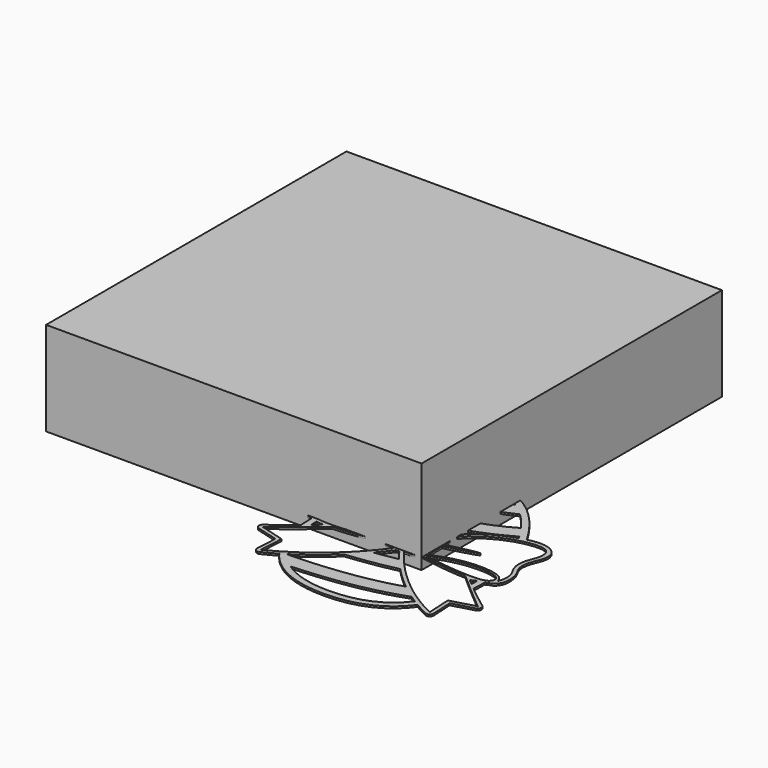
from build123d import *

# Parameters (mm, degrees)
F0_W     = 100
F0_H     = 100
F1_DEPTH = 25
F3_DEPTH = 5
F4_SCALE = 0.1


with BuildPart() as f1:
    # F0 (on Top) → F1 (new body)
    with BuildSketch(Plane.XY):
        with Locations((-50, 50)):
            Rectangle(F0_W, F0_H)
    extrude(amount=F1_DEPTH)


with BuildPart() as f3:
    # F2 (on face) → F3 (new body)
    with BuildSketch(Plane.XY.offset(25)):
        Polygon((237.0909, -93.2355584012), (234.964781, -91.1346954012), (230.904136, -88.1422674012), (225.837062, -84.3918364012), (219.722472, -79.8171774012), (212.519281, -74.3520704012), (204.186402, -67.9302914012), (194.68275, -60.4856174012), (183.967238, -51.9518264012), (171.998781, -42.2626954012), (172.36901, -37.8418454012), (172.685672, -33.4080234012), (172.949107, -28.9619434012), (173.159656, -24.5043204012), (173.317658, -20.0358694012), (173.423453, -15.5573044012), (173.477381, -11.0693414012), (173.479781, -6.5726954012), (174.402898, -6.2096524012), (175.317906, -5.8351014012), (176.224289, -5.4476604012), (177.121531, -5.0459454012), (178.009117, -4.6285744012), (178.886531, -4.1941644012), (179.753258, -3.7413324012), (180.608781, -3.2686954012), (182.202781, -2.6213224012), (184.271343, -2.0135234012), (186.723437, -1.2204044012), (189.468031, -0.0170704012), (192.414094, 1.8213725988), (195.470593, 4.5198205988), (198.5465, 8.3031655988), (201.550781, 13.3963045988), (202.989537, 16.5327435988), (204.06814, 19.5250075988), (204.83847, 22.4765135988), (205.352406, 25.4906795988), (205.661826, 28.6709235988), (205.818609, 32.1206635988), (205.874635, 35.9433185988), (205.881781, 40.2423045988), (204.442482, 53.2482925988), (201.031328, 63.6247105988), (196.627056, 72.4642385988), (192.208406, 80.8595545988), (188.754115, 89.9033395988), (187.242922, 100.6882735988), (188.653564, 114.3070345988), (193.964781, 131.8523045988), (196.39601, 137.7646815988), (199.286672, 144.9972575988), (201.940732, 153.1809505988), (203.662156, 161.9466795988), (203.754908, 170.9253615988), (201.522953, 179.7479135988), (196.270256, 188.0452555988), (187.300781, 195.4483045988), (180.359689, 198.9783925988), (172.853109, 201.4293825988), (164.869459, 202.8953655988), (156.497156, 203.4704295988), (147.824619, 203.2486655988), (138.940265, 202.3241635988), (129.932513, 200.7910135988), (120.889781, 198.7433045988), (117.827379, 204.0665255988), (114.587812, 209.4891325988), (111.207293, 214.9619195988), (107.722031, 220.4356795988), (104.168238, 225.8612045988), (100.582125, 231.1892885988), (96.999902, 236.3707245988), (93.457781, 241.3563045988), (88.759427, 247.7524355988), (84.021078, 253.9551015988), (79.243424, 259.9650875988), (74.427156, 265.7831795988), (69.572967, 271.4101615988), (64.681547, 276.8468205988), (59.753588, 282.0939395988), (54.789781, 287.1523045988), (50.867982, 290.9924065988), (46.925078, 294.7163045988), (42.961056, 298.3226405988), (38.975906, 301.8100545988), (34.969615, 305.1771875988), (30.942172, 308.4226795988), (26.893564, 311.5451715988), (22.823781, 314.5433045988), (20.510547, 316.1929065988), (18.192719, 317.8138675988), (15.869734, 319.4026715988), (13.541031, 320.9558045988), (11.206047, 322.4697495988), (8.864218, 323.9409915988), (6.514984, 325.3660155988), (4.157781, 326.7413045988), (-6.978416, 332.6333945988), (-17.272235, 337.2170855988), (-26.657639, 340.6535115988), (-35.068594, 343.1038045988), (-42.439065, 344.7290975988), (-48.703016, 345.6905235988), (-53.794412, 346.1492145988), (-57.647219, 346.2663045988), (-57.713219, 346.2663045988), (-59.201219, 346.1993045988), (-59.308598, 346.2078685988), (-59.443375, 346.2173825988), (-59.605762, 346.2272005988), (-59.795969, 346.2366795988), (-60.014207, 346.2451735988), (-60.260688, 346.2520385988), (-60.535621, 346.2566305988), (-60.839219, 346.2583045988), (-66.458862, 345.9096425988), (-76.83436, 344.2184455988), (-91.353069, 340.1628965988), (-109.402344, 332.7211795988), (-130.369541, 320.8714785988), (-153.642016, 303.5919765988), (-178.607123, 279.8608575988), (-204.652219, 248.6563045988), (-208.25103, 243.7714135988), (-211.856953, 238.7293045988), (-215.468479, 233.5263205988), (-219.084094, 228.1588045988), (-222.702287, 222.6231015988), (-226.321547, 216.9155545988), (-229.940362, 211.0325075988), (-233.557219, 204.9703045988), (-233.563133, 204.9601385988), (-233.568906, 204.9499135988), (-233.574586, 204.9396655988), (-233.580219, 204.9294295988), (-233.585852, 204.9192405988), (-233.591532, 204.9091325988), (-233.597305, 204.8991425988), (-233.603219, 204.8893045988), (-234.068307, 204.0859335988), (-234.527735, 203.2726485988), (-234.982873, 202.4518165988), (-235.435094, 201.6258045988), (-235.885768, 200.7969805988), (-236.336266, 199.9677105988), (-236.787959, 199.1403635988), (-237.242219, 198.3173045988), (-259.482606, 202.2216225988), (-278.47575, 202.8087265988), (-293.944504, 199.9925875988), (-305.611719, 193.6871795988), (-313.200246, 183.8064745988), (-316.432938, 170.2644455988), (-315.032645, 152.9750645988), (-308.722219, 131.8523045988), (-303.338485, 114.1410445988), (-301.893469, 100.4904135988), (-303.399703, 89.7643845988), (-306.869719, 80.8269295988), (-311.316047, 72.5420215988), (-315.751219, 63.7736325988), (-319.187766, 53.3857365988), (-320.638219, 40.2423045988), (-320.631115, 35.9433185988), (-320.575203, 32.1206635988), (-320.41858, 28.6709235988), (-320.109344, 25.4906795988), (-319.595592, 22.4765135988), (-318.825422, 19.5250075988), (-317.746932, 16.5327435988), (-316.308219, 13.3963045988), (-313.303938, 8.3031655988), (-310.228032, 4.5198205988), (-307.171532, 1.8213725988), (-304.225469, -0.0170704012), (-301.480875, -1.2204044012), (-299.028782, -2.0135234012), (-296.960219, -2.6213224012), (-295.366219, -3.2686954012), (-294.517119, -3.7377204012), (-293.656922, -4.1872114012), (-292.786155, -4.6185374012), (-291.905344, -5.0330704012), (-291.015018, -5.4321814012), (-290.115703, -5.8172424012), (-289.207928, -6.1896234012), (-288.292219, -6.5506954012), (-288.267297, -11.0404204012), (-288.195219, -15.5230544012), (-288.074391, -19.9974164012), (-287.903219, -24.4623204012), (-287.68011, -28.9165844012), (-287.403469, -33.3590234012), (-287.071703, -37.7884554012), (-286.683219, -42.2036954012), (-295.865451, -49.6504184012), (-304.444766, -56.5207894012), (-312.399963, -62.8121134012), (-319.709844, -68.5216954012), (-326.353209, -73.6468404012), (-332.30886, -78.1848514012), (-337.555596, -82.1330354012), (-342.072219, -85.4886954012), (-349.722219, -91.1346954012), (-350.809826, -92.0626684012), (-351.741891, -93.1185394012), (-352.510901, -94.2831134012), (-353.109344, -95.5371954012), (-353.529709, -96.8615904012), (-353.764485, -98.2371014012), (-353.806158, -99.6445354012), (-353.647219, -101.0646954012), (-353.289108, -102.4490214012), (-352.748266, -103.7494294012), (-352.038557, -104.9508144012), (-351.173844, -106.0380704012), (-350.16799, -106.9960914012), (-349.03486, -107.8097734012), (-347.788315, -108.4640094012), (-346.442219, -108.9436954012), (-289.381219, -124.8146954012), (-292.504219, -181.5086954012), (-292.489408, -182.8403474012), (-292.302297, -184.1417894012), (-291.95049, -185.3979964012), (-291.441594, -186.5939454012), (-290.783213, -187.7146134012), (-289.982953, -188.7449764012), (-289.04842, -189.6700114012), (-287.987219, -190.4746954012), (-286.831637, -191.1303674012), (-285.615375, -191.6233834012), (-284.35491, -191.9522424012), (-283.066719, -192.1154454012), (-281.767278, -192.1114924012), (-280.473063, -191.9388824012), (-279.200551, -191.5961174012), (-277.966219, -191.0816954012), (-270.834219, -187.5406954012), (-267.059401, -185.6385254012), (-263.32186, -183.7060864012), (-259.619217, -181.7457324012), (-255.949094, -179.7598204012), (-252.309112, -177.7507054012), (-248.696891, -175.7207424012), (-245.110053, -173.6722874012), (-241.546219, -171.6076954012), (-238.360342, -175.9037384012), (-235.086891, -180.0914764012), (-231.724635, -184.1691994012), (-228.272344, -188.1351954012), (-224.728787, -191.9877544012), (-221.092735, -195.7251644012), (-217.362955, -199.3457154012), (-213.538219, -202.8476954012), (-198.399018, -214.9473224012), (-182.00011, -225.4533984012), (-164.347787, -234.3598414012), (-145.448344, -241.6605704012), (-125.308073, -247.3495024012), (-103.933266, -251.4205544012), (-81.330217, -253.8676464012), (-57.505219, -254.6846954012), (-57.339446, -254.6845234012), (-57.172407, -254.6840704012), (-57.004524, -254.6834294012), (-56.836219, -254.6826954012), (-56.667914, -254.6819614012), (-56.500031, -254.6813204012), (-56.332992, -254.6808674012), (-56.167219, -254.6806954012), (-26.238758, -253.2771544012), (1.721281, -249.2984294012), (27.698508, -242.7548694012), (51.678531, -233.6568204012), (73.646961, -222.0146314012), (93.589406, -207.8386484012), (111.491476, -191.1392204012), (127.338781, -171.9266954012), (130.837927, -173.9488284012), (134.358953, -175.9554454012), (137.904236, -177.9442504012), (141.476156, -179.9129454012), (145.077092, -181.8592344012), (148.709422, -183.7808204012), (152.375525, -185.6754064012), (156.077781, -187.5406954012), (158.654748, -188.8302574012), (160.708015, -189.8633204012), (162.338635, -190.6659454012), (163.647656, -191.2641954012), (164.736131, -191.6841324012), (165.705109, -191.9518204012), (166.655642, -192.0933204012), (167.688781, -192.1346954012), (169.796326, -191.9141544012), (171.747578, -191.2836794012), (173.499213, -190.2899944012), (175.007906, -188.9798204012), (176.230334, -187.3998814012), (177.123172, -185.5968984012), (177.643095, -183.6175954012), (177.746781, -181.5086954012), (174.623781, -124.8146954012), (231.684781, -108.9436954012), (234.419834, -107.7373004012), (236.55089, -105.9124144012), (238.047799, -103.6326054012), (238.880406, -101.0614454012), (239.01856, -98.3625044012), (238.432109, -95.6993514012), align=None)
        Polygon((-213.538166, -163.7059244012), (-226.120219, -163.9726954012), (-226.22711, -163.8281644012), (-226.332782, -163.6821334012), (-226.43761, -163.5350704012), (-226.541969, -163.3874454012), (-226.646235, -163.2397264012), (-226.750781, -163.0923824012), (-226.855985, -162.9458824012), (-226.962219, -162.8006954012), (-213.694973, -154.1968044012), (-200.903438, -145.3704454012), (-188.589418, -136.3633364012), (-176.754719, -127.2171954012), (-165.401145, -117.9737424012), (-154.5305, -108.6746954012), (-144.14459, -99.3617734012), (-134.245219, -90.0766954012), (-117.462369, -88.1774144012), (-100.879735, -86.1223204012), (-84.432311, -83.8765394012), (-68.055094, -81.4051954012), (-51.68308, -78.6734144012), (-35.251266, -75.6463204012), (-18.694647, -72.2890394012), (-1.948219, -68.5666954012), (4.463271, -75.2271754012), (11.14489, -81.9646014012), (18.095361, -88.7624494012), (25.313406, -95.6041954012), (32.797748, -102.4733164012), (40.547109, -109.3532894012), (48.560213, -116.2275904012), (56.835781, -123.0796954012), (34.486791, -129.8617164012), (11.872172, -135.8481174012), (-10.944924, -141.0949004012), (-33.901344, -145.6580704012), (-56.933936, -149.5936314012), (-79.979547, -152.9575864012), (-102.975026, -155.8059394012), (-125.857219, -158.1946954012), (-138.303756, -159.3313264012), (-150.785578, -160.3613044012), (-163.297377, -161.2787594012), (-175.833844, -162.0778204012), (-188.38967, -162.7526154012), (-200.959547, -163.2972734012), align=None, mode=Mode.SUBTRACT)
        Polygon((-250.422615, -164.8650254012), (-282.446219, -182.0626954012), (-278.877219, -117.2816954012), (-343.742219, -99.2386954012), (-336.092219, -93.5936954012), (-331.863619, -90.4538944012), (-326.993922, -86.7951644012), (-321.50053, -82.6196364012), (-315.400844, -77.9294454012), (-308.712268, -72.7267224012), (-301.452203, -67.0136014012), (-293.638053, -60.7922154012), (-285.287219, -54.0646954012), (-283.42328, -52.5518904012), (-281.536266, -51.0162584012), (-279.625885, -49.4574684012), (-277.691844, -47.8751954012), (-275.73385, -46.2691094012), (-273.75161, -44.6388824012), (-271.74483, -42.9841874012), (-269.713219, -41.3046954012), (-265.33074, -37.6675644012), (-260.851828, -33.9304614012), (-256.275393, -30.0908184012), (-251.600344, -26.1460704012), (-246.825592, -22.0936504012), (-241.950047, -17.9309924012), (-236.972619, -13.6555294012), (-231.892219, -9.2646954012), (-230.654219, -8.1916954012), (-229.018219, -8.1326954012), (-217.499412, -7.5731314012), (-205.040141, -6.6661174012), (-191.573877, -5.4036744012), (-177.034094, -3.7778204012), (-161.354264, -1.7805764012), (-144.46786, 0.5960385988), (-126.308354, 3.3600055988), (-106.809219, 6.5193045988), (-104.538418, 4.5635345988), (-102.094438, 2.8193355988), (-99.49141, 1.3018705988), (-96.743469, 0.0263045988), (-93.864746, -0.9921994012), (-90.869375, -1.7384764012), (-87.771489, -2.1973634012), (-84.585219, -2.3536954012), (-70.368219, -2.3536954012), (-91.423588, -29.4072564012), (-114.02036, -55.3425544012), (-138.16703, -80.0630174012), (-163.872094, -103.4720704012), (-191.144049, -125.4731384012), (-219.991391, -145.9696484012), align=None, mode=Mode.SUBTRACT)
        Polygon((-271.381963, -13.0051934012), (-271.421219, -10.7076954012), (-269.065772, -11.0070584012), (-266.648203, -11.2681014012), (-264.165549, -11.4926294012), (-261.614844, -11.6824454012), (-258.993123, -11.8393554012), (-256.297422, -11.9651644012), (-253.524776, -12.0616754012), (-250.672219, -12.1306954012), (-253.284994, -14.3593384012), (-255.860797, -16.5479614012), (-258.402217, -18.6994824012), (-260.911844, -20.8168204012), (-263.392268, -22.9028924012), (-265.846078, -24.9606174012), (-268.275865, -26.9929124012), (-270.684219, -29.0026954012), (-270.824209, -26.7258694012), (-270.951953, -24.4463364012), (-271.066737, -22.1640134012), (-271.167844, -19.8788204012), (-271.254561, -17.5906744012), (-271.326172, -15.2994924012), align=None, mode=Mode.SUBTRACT)
        Polygon((-290.121455, 5.3401565988), (-290.392219, 5.4893045988), (-292.844405, 7.3426695988), (-294.901516, 9.9026635988), (-296.34426, 12.9936345988), (-296.953344, 16.4399295988), (-296.509475, 20.0658965988), (-294.79336, 23.6958825988), (-291.585705, 27.1542365988), (-286.667219, 30.2653045988), (-279.19591, 32.9669495988), (-267.669375, 35.5063355988), (-252.506699, 37.3696445988), (-234.126969, 38.0430545988), (-212.94927, 37.0127455988), (-189.392688, 33.7648985988), (-163.876309, 27.7856915988), (-136.819219, 18.5613045988), (-136.398623, 18.3965895988), (-135.977078, 18.2352735988), (-135.554948, 18.0759725988), (-135.132594, 17.9173045988), (-134.710381, 17.7578865988), (-134.288672, 17.5963355988), (-133.86783, 17.4312695988), (-133.448219, 17.2613045988), (-118.066219, 10.9143045988), (-134.514219, 8.3983045988), (-151.345541, 5.9110995988), (-167.13611, 3.7631635988), (-181.909326, 1.9521425988), (-195.688594, 0.4756795988), (-208.497315, -0.6685804012), (-220.358891, -1.4829924012), (-231.296725, -1.9699124012), (-241.334219, -2.1316954012), (-242.348219, -2.1316954012), (-246.546055, -2.1137854012), (-250.567594, -2.0561014012), (-254.419258, -1.9527154012), (-258.107469, -1.7976954012), (-261.638649, -1.5851134012), (-265.019219, -1.3090394012), (-268.255602, -0.9635434012), (-271.354219, -0.5426954012), (-273.724311, -0.1478844012), (-276.011141, 0.3054135988), (-278.217791, 0.8196265988), (-280.347344, 1.3971795988), (-282.402881, 2.0404975988), (-284.387485, 2.7520075988), (-286.304237, 3.5341345988), (-288.156219, 4.3893045988), (-288.437155, 4.5246715988), (-288.719766, 4.6579295988), (-289.00301, 4.7904375988), (-289.285844, 4.9235545988), (-289.567225, 5.0586405988), (-289.84611, 5.1970545988), align=None, mode=Mode.SUBTRACT)
        Polygon((-52.548199, -8.2580024012), (-52.502219, -8.3226954012), (-50.269643, -11.3354294012), (-47.921485, -14.4585084012), (-45.45935, -17.6864924012), (-42.884844, -21.0139454012), (-40.199573, -24.4354294012), (-37.405141, -27.9455074012), (-34.503155, -31.5387424012), (-31.495219, -35.2096954012), (-39.067754, -36.7481334012), (-46.647438, -38.2186954012), (-54.232137, -39.6236324012), (-61.819719, -40.9651954012), (-69.408051, -42.2456334012), (-76.995, -43.4671954012), (-84.578434, -44.6321334012), (-92.156219, -45.7426954012), (-87.725184, -40.5492184012), (-83.488188, -35.4796324012), (-79.44727, -30.5457034012), (-75.604469, -25.7591954012), (-71.961824, -21.1318754012), (-68.521375, -16.6755074012), (-65.28516, -12.4018594012), (-62.255219, -8.3226954012), (-62.209239, -8.2580024012), (-62.165438, -8.1923364012), (-62.123278, -8.1259434012), (-62.082219, -8.0590704012), (-62.041723, -7.9919634012), (-62.00125, -7.9248674012), (-61.960262, -7.8580294012), (-61.918219, -7.7916954012), (-52.839219, -7.7916954012), (-52.797176, -7.8580294012), (-52.756188, -7.9248674012), (-52.715715, -7.9919634012), (-52.675219, -8.0590704012), (-52.63416, -8.1259434012), (-52.592, -8.1923364012), align=None, mode=Mode.SUBTRACT)
        Polygon((-28.661184, -236.3879124012), (-56.233219, -237.6536954012), (-56.391531, -237.6538674012), (-56.548719, -237.6543204012), (-56.705156, -237.6549614012), (-56.861219, -237.6556954012), (-57.017282, -237.6564294012), (-57.173719, -237.6570704012), (-57.330907, -237.6575234012), (-57.489219, -237.6576954012), (-76.768164, -237.0937134012), (-95.185031, -235.4053984012), (-112.735367, -232.5959514012), (-129.414719, -228.6685704012), (-145.218633, -223.6264554012), (-160.142656, -217.4728044012), (-174.182336, -210.2108184012), (-187.333219, -201.8436954012), (-178.836147, -201.3864334012), (-170.346141, -200.8726644012), (-161.864643, -200.3046604012), (-153.393094, -199.6846954012), (-144.932936, -199.0150434012), (-136.48561, -198.2979764012), (-128.052557, -197.5357694012), (-119.635219, -196.7306954012), (-92.691285, -193.8114334012), (-65.598125, -190.2697894012), (-38.451949, -186.0234724012), (-11.348969, -180.9901954012), (15.614605, -175.0876684012), (42.342562, -168.2336014012), (68.738691, -160.3457074012), (94.706781, -151.3416954012), (96.905418, -152.8366364012), (99.117625, -154.3244764012), (101.343472, -155.8052384012), (103.583031, -157.2789454012), (105.836371, -158.7456214012), (108.103562, -160.2052894012), (110.384676, -161.6579724012), (112.679781, -163.1036954012), (98.113308, -180.4092134012), (81.650437, -195.4517114012), (63.303988, -208.2217324012), (43.086781, -218.7098204012), (21.011636, -226.9065174012), (-2.908625, -232.8023674012), align=None, mode=Mode.SUBTRACT)
        Polygon((229.237781, -99.0986954012), (163.813781, -117.2816954012), (167.383781, -182.0676954012), (154.837015, -175.6883404012), (142.581906, -169.1448514012), (130.491234, -162.3109724012), (118.437781, -155.0604454012), (106.294328, -147.2670114012), (93.933656, -138.8044144012), (81.228547, -129.5463944012), (68.051781, -119.3666954012), (51.966461, -106.1299254012), (36.410031, -92.4023514012), (21.403164, -78.2308244012), (6.966531, -63.6621954012), (-6.879196, -48.7433164012), (-20.113344, -33.5210394012), (-32.715242, -18.0422154012), (-44.664219, -2.3536954012), (-29.920219, -2.3536954012), (-26.749377, -2.1988304012), (-23.66611, -1.7442114012), (-20.684303, -1.0048024012), (-17.817844, 0.0044295988), (-15.080619, 1.2685215988), (-12.486516, 2.7725075988), (-10.04942, 4.5014235988), (-7.783219, 6.4403045988), (3.956043, 4.5219415988), (15.218562, 2.7468985988), (26.019691, 1.1126205988), (36.374781, -0.3834454012), (46.299183, -1.7438554012), (55.80825, -2.9711644012), (64.917332, -4.0679254012), (73.641781, -5.0366954012), (80.447965, -5.7311174012), (87.018812, -6.3440704012), (93.357019, -6.8750864012), (99.465281, -7.3236954012), (105.346293, -7.6894294012), (111.00275, -7.9718204012), (116.437347, -8.1703984012), (121.652781, -8.2846954012), (123.371781, -8.3096954012), (139.960806, -22.9481014012), (155.274797, -36.3506954012), (169.471873, -48.6654144012), (182.710156, -60.0401954012), (195.147767, -70.6229764012), (206.942828, -80.5616954012), (218.253459, -90.0042894012), align=None, mode=Mode.SUBTRACT)
        Polygon((156.19326, -26.8342694012), (156.072781, -29.1246954012), (154.390545, -27.7205334012), (152.692828, -26.2998364012), (150.979994, -24.8630374012), (149.252406, -23.4105704012), (147.510427, -21.9428694012), (145.754422, -20.4603674012), (143.984752, -18.9634984012), (142.201781, -17.4526954012), (143.714607, -16.6683384012), (145.223953, -15.8777114012), (146.729994, -15.0811074012), (148.232906, -14.2788204012), (149.732865, -13.4711424012), (151.230047, -12.6583674012), (152.724627, -11.8407874012), (154.216781, -11.0186954012), (154.521558, -10.9830294012), (154.825375, -10.9465544012), (155.128207, -10.9093064012), (155.430031, -10.8713204012), (155.730824, -10.8326314012), (156.030562, -10.7932734012), (156.329222, -10.7532834012), (156.626781, -10.7126954012), (156.606381, -13.0241214012), (156.572703, -15.3330394012), (156.525408, -17.6392854012), (156.464156, -19.9426954012), (156.388607, -22.2431054012), (156.298422, -24.5403514012), align=None, mode=Mode.SUBTRACT)
        Polygon((176.532521, 6.1397885988), (173.311781, 3.7613045988), (165.659586, 0.8176175988), (155.562156, -1.0366954012), (143.787351, -1.9902574012), (131.103031, -2.2316954012), (118.277054, -1.9496334012), (106.077281, -1.3326954012), (95.27157, -0.5695074012), (86.627781, 0.1513045988), (78.900927, 0.8614375988), (70.981265, 1.6623675988), (62.869767, 2.5545155988), (54.567406, 3.5383045988), (46.075154, 4.6141565988), (37.393984, 5.7824915988), (28.524869, 7.0437345988), (19.468781, 8.3983045988), (3.031781, 10.9143045988), (18.399781, 17.2613045988), (44.972429, 26.6903805988), (70.361531, 32.9766635988), (94.09857, 36.5773615988), (115.715031, 37.9496795988), (134.742398, 37.5508255988), (150.712156, 35.8380075988), (163.155789, 33.2684315988), (171.604781, 30.2993045988), (176.419494, 27.2895075988), (179.586047, 23.8358045988), (181.271185, 20.1162265988), (181.641656, 16.3088045988), (180.864205, 12.5915705988), (179.105578, 9.1425545988), align=None, mode=Mode.SUBTRACT)
        Polygon((-304.305475, 19.5712535988), (-306.534219, 15.8383045988), (-306.675899, 16.4043885988), (-307.006907, 17.7262265988), (-307.463821, 19.5519475988), (-307.983219, 21.6296795988), (-308.50168, 23.7075525988), (-308.955781, 25.5336955988), (-309.282102, 26.8562365988), (-309.417219, 27.4233045988), (-310.574992, 40.2948965988), (-309.587719, 50.4231635988), (-307.052258, 58.6372205988), (-303.565469, 65.7661795988), (-299.724211, 72.6391545988), (-296.125344, 80.0852575988), (-293.365727, 88.9336035988), (-292.042219, 100.0133045988), (-292.003219, 102.7383045988), (-292.521256, 111.3432575988), (-293.915141, 118.9946795988), (-295.926533, 126.0110385988), (-298.297094, 132.7108045988), (-300.768483, 139.4124455988), (-303.08236, 146.4344295988), (-304.980385, 154.0952265988), (-306.204219, 162.7133045988), (-306.235385, 165.4608025988), (-305.879235, 168.5896635988), (-305.11267, 171.9646895988), (-303.912594, 175.4506795988), (-302.255908, 178.9124355988), (-300.119516, 182.2147575988), (-297.480319, 185.2224475988), (-294.315219, 187.8003045988), (-292.307158, 189.0129065988), (-290.109547, 190.0658045988), (-287.72474, 190.9583905988), (-285.155094, 191.6900545988), (-282.402963, 192.2601875988), (-279.470703, 192.6681795988), (-276.36067, 192.9134215988), (-273.075219, 192.9953045988), (-269.746692, 192.9274175988), (-266.244375, 192.7267105988), (-262.581043, 192.3976135988), (-258.769469, 191.9445545988), (-254.822426, 191.3719645988), (-250.752688, 190.6842735988), (-246.573028, 189.8859095988), (-242.296219, 188.9813045988), (-240.238053, 188.5164065988), (-238.162766, 188.0284915988), (-236.071049, 187.5176095988), (-233.963594, 186.9838045988), (-231.841092, 186.4271245988), (-229.704235, 185.8476165988), (-227.553713, 185.2453275988), (-225.390219, 184.6203045988), (-220.858985, 183.2524155988), (-216.297094, 181.7974455988), (-211.715141, 180.2571855988), (-207.123719, 178.6334295988), (-202.533422, 176.9279705988), (-197.954844, 175.1426015988), (-193.398578, 173.2791155988), (-188.875219, 171.3393045988), (-184.984959, 169.5942835988), (-181.200578, 167.8031955988), (-177.518924, 165.9705055988), (-173.936844, 164.1006795988), (-170.451186, 162.1981815988), (-167.058797, 160.2674765988), (-163.756526, 158.3130295988), (-160.541219, 156.3393045988), (-152.96501, 151.3917435988), (-145.573547, 146.1201955988), (-138.397826, 140.5353575988), (-131.468844, 134.6479295988), (-124.817596, 128.4686115988), (-118.475078, 122.0081015988), (-112.472287, 115.2770995988), (-106.840219, 108.2863045988), (-110.553975, 104.1833905988), (-113.245328, 100.0134915988), (-115.076783, 95.8404995988), (-116.210844, 91.7283045988), (-116.810014, 87.7407965988), (-117.036797, 83.9418665988), (-117.053698, 80.3954065988), (-117.023219, 77.1653045988), (-131.435196, 80.6040055988), (-144.773407, 83.6524135988), (-156.784024, 86.2596115988), (-167.213219, 88.3746795988), (-175.807164, 89.9467005988), (-182.312031, 90.9247575988), (-186.473992, 91.2579315988), (-188.039219, 90.8953045988), (-186.788049, 89.8160605988), (-182.83811, 88.1094765988), (-176.449381, 85.8537755988), (-167.881844, 83.1271795988), (-157.395479, 80.0079115988), (-145.250266, 76.5741955988), (-131.706186, 72.9042515988), (-117.023219, 69.0763045988), (-117.071791, 55.8504605988), (-117.152672, 45.3293045988), (-117.168608, 37.0708985988), (-117.022344, 30.6333045988), (-116.616627, 25.5745855988), (-115.854203, 21.4528045988), (-114.637819, 17.8260235988), (-112.870219, 14.2523045988), (-114.48934, 15.0336245988), (-116.099438, 15.7889295988), (-117.701989, 16.5224845988), (-119.298469, 17.2385545988), (-120.890356, 17.9414065988), (-122.479125, 18.6353045988), (-124.066254, 19.3245155988), (-125.653219, 20.0133045988), (-151.307692, 29.7648125988), (-176.186125, 36.7066795988), (-199.874918, 41.1525465988), (-221.960469, 43.4160545988), (-242.029176, 43.8108435988), (-259.667438, 42.6505545988), (-274.461653, 40.2488275988), (-285.998219, 36.9193045988), (-290.001135, 35.1669175988), (-293.280172, 33.2237735988), (-295.992139, 31.0591445988), (-298.293844, 28.6423045988), (-300.342096, 25.9425275988), (-302.293703, 22.9290855988), align=None, mode=Mode.SUBTRACT)
        Polygon((-219.058953, 196.0227045988), (-218.875219, 196.3403045988), (-217.982772, 197.8535405988), (-217.090453, 199.3550705988), (-216.198299, 200.8449975988), (-215.306344, 202.3234295988), (-214.414623, 203.7904705988), (-213.523172, 205.2462265988), (-212.632026, 206.6908025988), (-211.741219, 208.1243045988), (-202.319453, 209.6564235988), (-192.912781, 211.2614455988), (-183.523266, 212.9366155988), (-174.152969, 214.6791795988), (-164.803953, 216.4863845988), (-155.478281, 218.3554765988), (-146.178016, 220.2837005988), (-136.905219, 222.2683045988), (-114.608981, 227.3360795988), (-92.275125, 232.8980705988), (-69.971692, 239.0002715988), (-47.766719, 245.6886795988), (-25.728246, 253.0092905988), (-3.924313, 261.0081015988), (17.577043, 269.7311075988), (38.707781, 279.2243045988), (43.871033, 274.1549195988), (48.997734, 268.8589765988), (54.087427, 263.3379155988), (59.139656, 257.5931795988), (64.153963, 251.6262085988), (69.12989, 245.4384455988), (74.066982, 239.0313295988), (78.964781, 232.4063045988), (52.930605, 218.3229495988), (25.909312, 205.9363985988), (-1.902996, 195.0959255988), (-30.310219, 185.6508045988), (-59.116254, 177.4503085988), (-88.125, 170.3437105988), (-117.140356, 164.1802845988), (-145.966219, 158.8093045988), (-150.187278, 161.6748085988), (-154.582688, 164.5198985988), (-159.156176, 167.3338165988), (-163.911469, 170.1058045988), (-168.852293, 172.8251055988), (-173.982375, 175.4809605988), (-179.305442, 178.0626135988), (-184.825219, 180.5593045988), (-189.033014, 182.3717065988), (-193.327328, 184.1499605988), (-197.697557, 185.8877615988), (-202.133094, 187.5788045988), (-206.623334, 189.2167845988), (-211.157672, 190.7953985988), (-215.725502, 192.3083395988), (-220.316219, 193.7493045988), (-220.134453, 194.0705135988), (-219.954656, 194.3950385988), (-219.776078, 194.7216035988), (-219.597969, 195.0489295988), (-219.419578, 195.3757405988), (-219.240157, 195.7007575988), align=None, mode=Mode.SUBTRACT)
        Polygon((-65.357471, 328.9524115988), (-60.789219, 329.2313045988), (-60.336631, 329.2059005988), (-59.943328, 329.1910075988), (-59.584502, 329.1852325988), (-59.235344, 329.1871795988), (-58.871045, 329.1954545988), (-58.466797, 329.2086635988), (-57.997791, 329.2254115988), (-57.439219, 329.2443045988), (-57.414219, 329.2443045988), (-54.729115, 329.1590295988), (-50.773641, 328.7976015988), (-45.618049, 328.0016185988), (-39.332594, 326.6126795988), (-31.98753, 324.4723805988), (-23.65311, 321.4223205988), (-14.399588, 317.3040955988), (-4.297219, 311.9593045988), (-3.182531, 311.3086505988), (-2.070844, 310.6353205988), (-0.961594, 309.9436385988), (0.145781, 309.2379295988), (1.251844, 308.5225175988), (2.357156, 307.8017265988), (3.462281, 307.0798805988), (4.567781, 306.3613045988), (-13.930274, 298.8216285988), (-32.682531, 291.8628985988), (-51.631383, 285.4439335988), (-70.719219, 279.5235545988), (-89.88843, 274.0605815988), (-109.081407, 269.0138355988), (-128.240539, 264.3421365988), (-147.308219, 260.0043045988), (-151.354836, 259.1202065988), (-155.389407, 258.2523985988), (-159.413008, 257.4001055988), (-163.426719, 256.5625545988), (-167.431617, 255.7389725988), (-171.428782, 254.9285855988), (-175.419289, 254.1306205988), (-179.404219, 253.3443045988), (-157.285545, 277.5530255988), (-136.402578, 295.9792575988), (-117.179151, 309.4109825988), (-100.039094, 318.6361795988), (-85.40624, 324.4428295988), (-73.704422, 327.6189135988), align=None, mode=Mode.SUBTRACT)
        Polygon((-33.971219, 4.7993045988), (-80.484219, 4.7993045988), (-86.281405, 5.4473475988), (-91.628391, 7.2909605988), (-96.425698, 10.1793705988), (-100.573844, 13.9618045988), (-103.97335, 18.4874885988), (-106.524735, 23.6056485988), (-108.128518, 29.1655115988), (-108.685219, 35.0163045988), (-108.685219, 84.8553045988), (-108.10961, 90.9251615988), (-106.459906, 96.5878515988), (-103.851797, 101.7194235988), (-100.400969, 106.1959295988), (-96.22311, 109.8934195988), (-91.433906, 112.6879455988), (-86.149047, 114.4555565988), (-80.484219, 115.0723045988), (-33.971219, 115.0723045988), (-28.244088, 114.4424315988), (-22.929985, 112.6429455988), (-18.136967, 109.8090445988), (-13.973094, 106.0759295988), (-10.546424, 101.5787985988), (-7.965016, 96.4528515988), (-6.336928, 90.8332865988), (-5.770219, 84.8553045988), (-5.770219, 35.0163045988), (-6.345787, 28.9461595988), (-7.995391, 23.2833355988), (-10.603377, 18.1517455988), (-14.054094, 13.6753045988), (-18.231889, 9.9779255988), (-23.02111, 7.1835235988), (-28.306104, 5.4160115988), align=None, mode=Mode.SUBTRACT)
        Polygon((75.987851, 186.8676035988), (100.277781, 200.2593045988), (100.58209, 199.7550725988), (101.025687, 199.0146955988), (101.563832, 198.1132795988), (102.151781, 197.1259295988), (102.744793, 196.1277515988), (103.298125, 195.1938515988), (103.767035, 194.3993335988), (104.106781, 193.8193045988), (88.873697, 188.4340035988), (74.140734, 182.4581485988), (59.921826, 175.8100585988), (46.230906, 168.4080545988), (33.081908, 160.1704565988), (20.488765, 151.0155855988), (8.465412, 140.8617615988), (-2.974219, 129.6273045988), (-4.293578, 128.2146635988), (-5.599906, 126.7792415988), (-6.893578, 125.3229135988), (-8.174969, 123.8475545988), (-9.444453, 122.3550385988), (-10.702406, 120.8472415988), (-11.949203, 119.3260385988), (-13.185219, 117.7933045988), (-15.356547, 118.8852695988), (-17.599782, 119.8478355988), (-19.910047, 120.6760115988), (-22.282469, 121.3648045988), (-24.712172, 121.9092225988), (-27.194281, 122.3042735988), (-29.723922, 122.5449645988), (-32.296219, 122.6263045988), (-50.119471, 122.6750665988), (-64.007485, 122.7503355988), (-74.618772, 122.7455895988), (-82.611844, 122.5543045988), (-88.645213, 122.0699565988), (-93.377391, 121.1860235988), (-97.466889, 119.7959805988), (-101.572219, 117.7933045988), (-102.435258, 118.8566155988), (-103.309407, 119.9060385988), (-104.192836, 120.9438145988), (-105.083719, 121.9721795988), (-105.980227, 122.9933725988), (-106.880532, 124.0096325988), (-107.782805, 125.0231975988), (-108.685219, 126.0363045988), (-81.501883, 131.8138655988), (-54.402969, 138.4162265988), (-27.498117, 145.9310335988), (-0.896969, 154.4459295988), (25.290836, 164.0485605988), (50.955656, 174.8265705988), align=None, mode=Mode.SUBTRACT)
        Polygon((167.172814, 191.8879475988), (179.061781, 188.4363045988), (182.378367, 186.0543495988), (185.061344, 183.4330385988), (187.169164, 180.5889545988), (188.760281, 177.5386795988), (189.893148, 174.2987945988), (190.626219, 170.8858825988), (191.017945, 167.3165255988), (191.126781, 163.6073045988), (190.503797, 156.0092245988), (188.839719, 148.8859765988), (186.491359, 141.9570485988), (183.815531, 134.9419295988), (181.169047, 127.5601075988), (178.908718, 119.5310705988), (177.391359, 110.5743065988), (176.973781, 100.4093045988), (178.017767, 90.8321695988), (180.213859, 82.9117265988), (183.167381, 76.1236655988), (186.483656, 69.9436795988), (189.76801, 63.8474585988), (192.625765, 57.3106955988), (194.662248, 49.8090795988), (195.482781, 40.8183045988), (195.402957, 37.0252185988), (195.170062, 33.6962425988), (194.793965, 30.6892965988), (194.284531, 27.8623045988), (193.651629, 25.0731875988), (192.905125, 22.1798665988), (192.054886, 19.0402655988), (191.110781, 15.5123045988), (189.24316, 19.1407025988), (187.512062, 22.4964295988), (185.754761, 25.5892815988), (183.808531, 28.4290545988), (181.510644, 31.0255465988), (178.698375, 33.3885545988), (175.208996, 35.5278745988), (170.879781, 37.4533045988), (160.940635, 40.3313595988), (146.746984, 42.7691165988), (128.775513, 44.1805935988), (107.502906, 43.9798045988), (83.405845, 41.5807655988), (56.961015, 36.3974915988), (28.645099, 27.8439995988), (-1.065219, 15.3343045988), (0.352636, 18.3266615988), (1.351875, 21.2261015988), (2.003254, 24.5630485988), (2.377531, 28.8679295988), (2.545465, 34.6711695988), (2.577812, 42.5031955988), (2.545332, 52.8944315988), (2.518781, 66.3753045988), (2.582074, 66.3910745988), (2.748937, 66.4326485988), (2.984847, 66.4914255988), (3.255281, 66.5588045988), (3.525715, 66.6261835988), (3.761625, 66.6849605988), (3.928488, 66.7265345988), (3.991781, 66.7423045988), (20.337039, 70.9145835988), (35.523218, 74.9516635988), (49.227679, 78.7564085988), (61.127781, 82.2316795988), (70.900883, 85.2803415988), (78.224344, 87.8052575988), (82.775523, 89.7092905988), (84.231781, 90.8953045988), (82.399773, 91.2560215988), (77.518593, 90.7979135988), (69.915383, 89.5865955988), (59.917281, 87.6876795988), (47.851429, 85.1667795988), (34.044968, 82.0895075988), (18.825039, 78.5214785988), (2.518781, 74.5283045988), (2.547101, 78.5729175988), (2.519593, 82.7983985988), (2.267554, 87.1490815988), (1.622281, 91.5693045988), (0.41507, 96.0034025988), (-1.522782, 100.3957105988), (-4.359977, 104.6905665988), (-8.265219, 108.8323045988), (15.259388, 134.1792085988), (42.015265, 154.5573515988), (70.371244, 170.2516265988), (98.696156, 181.5469295988), (125.358834, 188.7281545988), (148.728109, 192.0801955988), align=None, mode=Mode.SUBTRACT)
    extrude(amount=F3_DEPTH)


with BuildPart() as f3_1:
    # F4: moved
    add(f3.part.scale(F4_SCALE))


solid = Compound([f1.part, f3_1.part])
